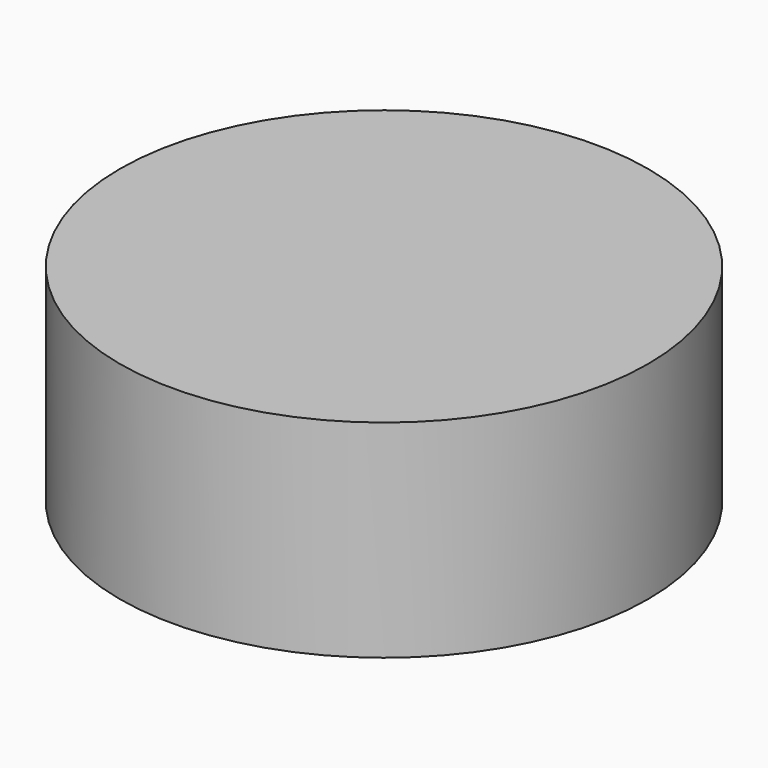
from build123d import *

# Parameters (mm, degrees)
F0_R = 63.5
F2_R = 63.5


with BuildPart() as f4:
    # F0 (on Top) → F4 section 0
    with BuildSketch(Plane.XY):
        Circle(F0_R)
    # F2 (on offset) → F4 section 1
    with BuildSketch(Plane.XY.offset(49.784)):
        Circle(F2_R)
    loft()


solid = f4.part
